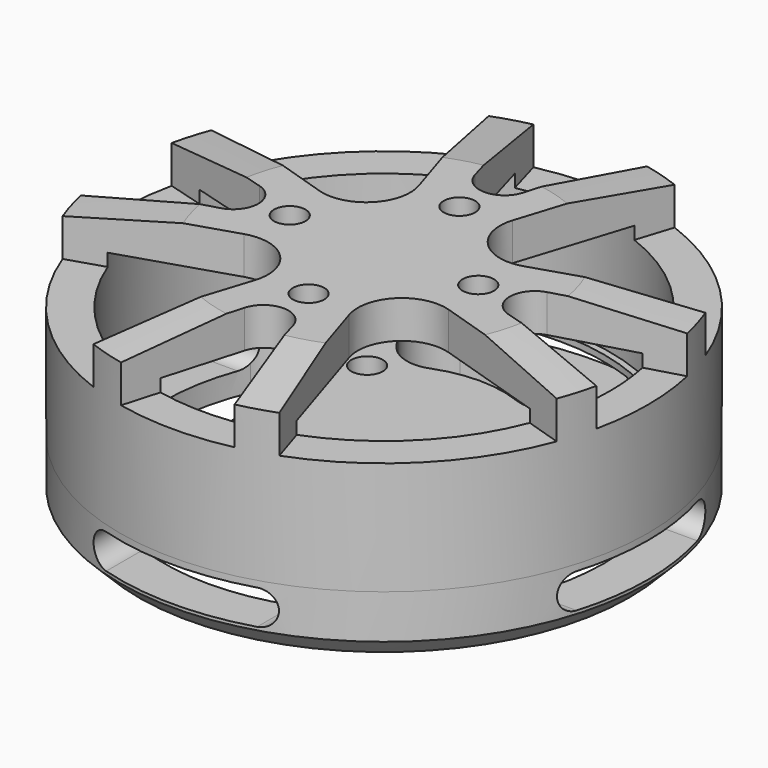
from build123d import *

# Parameters (mm, degrees)
F0_R            = 21
F1_DEPTH        = 5
F3_DEPTH        = 5.001
F4_SIZE         = 1.5
F7_DEPTH        = 10
F7_COPIES_COUNT = 4
F8_DEPTH        = 13
F10_DEPTH       = 4
F11_SIZE2       = 8
F11_SIZE        = 1
F12_R           = 18
F13_DEPTH       = 10
F15_D           = 2.5
F17_D           = 2.5


# Not quite as in the source:
# - a pattern or mirror of a feature is missing from the dataset's text; its kind, count and spacing are read off the source's solid


with BuildPart() as f1:
    # F0 (on Top) → F1 (new body)
    with BuildSketch(Plane.XY):
        Circle(F0_R)
    extrude(amount=-F1_DEPTH)

    # F2 (on face) → F3 (cut, through all)
    with BuildSketch(Plane.XY):
        with BuildLine():
            ThreePointArc((-3.4220516481, 8.8622549342), (0, 9.5), (3.4220516481, 8.8622549342))
            ThreePointArc((3.4220516481, 8.8622549342), (5.3769736461, 8.7910804429), (6.9601556698, 9.9401324464))
            Line((6.9601556698, 9.9401324464), (8.1369050061, 11.6207046655))
            ThreePointArc((8.1369050061, 11.6207046655), (8.5636626177, 14.1668496736), (6.8545072608, 16.1017306589))
            ThreePointArc((6.8545072608, 16.1017306589), (0, 17.5), (-6.8545072608, 16.1017306589))
            ThreePointArc((-6.8545072608, 16.1017306589), (-8.5636626177, 14.1668496736), (-8.1369050061, 11.6207046655))
            Line((-8.1369050061, 11.6207046655), (-6.9601556698, 9.9401324464))
            ThreePointArc((-6.9601556698, 9.9401324464), (-5.3769736461, 8.7910804429), (-3.4220516481, 8.8622549342))
        make_face()
        with BuildLine():
            ThreePointArc((-11.6207046655, 8.1369050061), (-14.1668496736, 8.5636626177), (-16.1017306589, 6.8545072608))
            ThreePointArc((-16.1017306589, 6.8545072608), (-17.5, 0), (-16.1017306589, -6.8545072608))
            ThreePointArc((-16.1017306589, -6.8545072608), (-14.1668496736, -8.5636626177), (-11.6207046655, -8.1369050061))
            Line((-11.6207046655, -8.1369050061), (-9.9401324464, -6.9601556698))
            ThreePointArc((-9.9401324464, -6.9601556698), (-8.7910804429, -5.3769736461), (-8.8622549342, -3.4220516481))
            ThreePointArc((-8.8622549342, -3.4220516481), (-9.5, 0), (-8.8622549342, 3.4220516481))
            ThreePointArc((-8.8622549342, 3.4220516481), (-8.7910804429, 5.3769736461), (-9.9401324464, 6.9601556698))
            Line((-9.9401324464, 6.9601556698), (-11.6207046655, 8.1369050061))
        make_face()
        with BuildLine():
            ThreePointArc((-8.1369050061, -11.6207046655), (-8.5636626177, -14.1668496736), (-6.8545072608, -16.1017306589))
            ThreePointArc((-6.8545072608, -16.1017306589), (0, -17.5), (6.8545072608, -16.1017306589))
            ThreePointArc((6.8545072608, -16.1017306589), (8.5636626177, -14.1668496736), (8.1369050061, -11.6207046655))
            Line((8.1369050061, -11.6207046655), (6.9601556698, -9.9401324464))
            ThreePointArc((6.9601556698, -9.9401324464), (5.3769736461, -8.7910804429), (3.4220516481, -8.8622549342))
            ThreePointArc((3.4220516481, -8.8622549342), (0, -9.5), (-3.4220516481, -8.8622549342))
            ThreePointArc((-3.4220516481, -8.8622549342), (-5.3769736461, -8.7910804429), (-6.9601556698, -9.9401324464))
            Line((-6.9601556698, -9.9401324464), (-8.1369050061, -11.6207046655))
        make_face()
        with BuildLine():
            ThreePointArc((11.6207046655, -8.1369050061), (14.1668496736, -8.5636626177), (16.1017306589, -6.8545072608))
            ThreePointArc((16.1017306589, -6.8545072608), (17.5, 0), (16.1017306589, 6.8545072608))
            ThreePointArc((16.1017306589, 6.8545072608), (14.1668496736, 8.5636626177), (11.6207046655, 8.1369050061))
            Line((11.6207046655, 8.1369050061), (9.9401324464, 6.9601556698))
            ThreePointArc((9.9401324464, 6.9601556698), (8.7910804429, 5.3769736461), (8.8622549342, 3.4220516481))
            ThreePointArc((8.8622549342, 3.4220516481), (9.5, 0), (8.8622549342, -3.4220516481))
            ThreePointArc((8.8622549342, -3.4220516481), (8.7910804429, -5.3769736461), (9.9401324464, -6.9601556698))
            Line((9.9401324464, -6.9601556698), (11.6207046655, -8.1369050061))
        make_face()
    extrude(amount=-F3_DEPTH, mode=Mode.SUBTRACT)

    # F4
    f4_edges = [f1.edges().sort_by_distance(p)[0] for p in [
        (-21, 0, -5),
    ]]
    chamfer(f4_edges, length=F4_SIZE)

    # F6 (on offset) → F7 (cut)
    with BuildSketch(Plane.XZ.offset(25)):
        with BuildLine():
            Line((6, -0.5), (-6, -0.5))
            ThreePointArc((-6, -0.5), (-7.375, -1.875), (-6, -3.25))
            Line((-6, -3.25), (6, -3.25))
            ThreePointArc((6, -3.25), (7.375, -1.875), (6, -0.5))
        make_face()
    f7 = extrude(amount=-F7_DEPTH, mode=Mode.SUBTRACT)

    # F7_copies: F7 ×4 about axis
    f7_copies_axis = Axis((0, 0, 0), (0, 0, 1))
    for i in range(1, F7_COPIES_COUNT):
        add(f7.rotate(f7_copies_axis, i * 360 / F7_COPIES_COUNT), mode=Mode.SUBTRACT)

    # F17 (through all)
    with Locations(Plane(origin=(0, 0, -5), x_dir=(1, 0, 0), z_dir=(0, 0, -1))):
        with Locations((-6.7175144213, -6.7175144213), (-8.8388347648, 8.8388347648), (6.7175144213, 6.7175144213), (8.8388347648, -8.8388347648)):
            Hole(F17_D / 2)


with BuildPart() as f8:
    # F0 (on Top) → F8 (new body)
    with BuildSketch(Plane.XY):
        Circle(F0_R)
    extrude(amount=F8_DEPTH)

    # F9 (on face) → F10 (cut)
    with BuildSketch(Plane.XY.offset(13)):
        with BuildLine():
            Line((-4.5201593688, 20.5077585143), (-1.9225233919, 11.4487252884))
            ThreePointArc((-1.9225233919, 11.4487252884), (0, 10), (1.9225233919, 11.4487252884))
            Line((1.9225233919, 11.4487252884), (4.5201593688, 20.5077585143))
            ThreePointArc((4.5201593688, 20.5077585143), (0, 21), (-4.5201593688, 20.5077585143))
        make_face()
        with BuildLine():
            Line((7.3962318513, 19.6544080145), (3.7353488919, 8.1307749821))
            ThreePointArc((3.7353488919, 8.1307749821), (4.5961940777, 4.5961940777), (8.1307749821, 3.7353488919))
            Line((8.1307749821, 3.7353488919), (19.6544080145, 7.3962318513))
            ThreePointArc((19.6544080145, 7.3962318513), (14.8492424049, 14.8492424049), (7.3962318513, 19.6544080145))
        make_face()
        with BuildLine():
            Line((-20.5077585143, -4.5201593688), (-11.4487252884, -1.9225233919))
            ThreePointArc((-11.4487252884, -1.9225233919), (-10, 0), (-11.4487252884, 1.9225233919))
            Line((-11.4487252884, 1.9225233919), (-20.5077585143, 4.5201593688))
            ThreePointArc((-20.5077585143, 4.5201593688), (-21, 0), (-20.5077585143, -4.5201593688))
        make_face()
        with BuildLine():
            Line((-19.6544080145, 7.3962318513), (-8.1307749821, 3.7353488919))
            ThreePointArc((-8.1307749821, 3.7353488919), (-4.5961940777, 4.5961940777), (-3.7353488919, 8.1307749821))
            Line((-3.7353488919, 8.1307749821), (-7.3962318513, 19.6544080145))
            ThreePointArc((-7.3962318513, 19.6544080145), (-14.8492424049, 14.8492424049), (-19.6544080145, 7.3962318513))
        make_face()
        with BuildLine():
            Line((4.5201593688, -20.5077585143), (1.9225233919, -11.4487252884))
            ThreePointArc((1.9225233919, -11.4487252884), (0, -10), (-1.9225233919, -11.4487252884))
            Line((-1.9225233919, -11.4487252884), (-4.5201593688, -20.5077585143))
            ThreePointArc((-4.5201593688, -20.5077585143), (0, -21), (4.5201593688, -20.5077585143))
        make_face()
        with BuildLine():
            Line((-7.3962318513, -19.6544080145), (-3.7353488919, -8.1307749821))
            ThreePointArc((-3.7353488919, -8.1307749821), (-4.5961940777, -4.5961940777), (-8.1307749821, -3.7353488919))
            Line((-8.1307749821, -3.7353488919), (-19.6544080145, -7.3962318513))
            ThreePointArc((-19.6544080145, -7.3962318513), (-14.8492424049, -14.8492424049), (-7.3962318513, -19.6544080145))
        make_face()
        with BuildLine():
            Line((20.5077585143, 4.5201593688), (11.4487252884, 1.9225233919))
            ThreePointArc((11.4487252884, 1.9225233919), (10, 0), (11.4487252884, -1.9225233919))
            Line((11.4487252884, -1.9225233919), (20.5077585143, -4.5201593688))
            ThreePointArc((20.5077585143, -4.5201593688), (21, 0), (20.5077585143, 4.5201593688))
        make_face()
        with BuildLine():
            Line((19.6544080145, -7.3962318513), (8.1307749821, -3.7353488919))
            ThreePointArc((8.1307749821, -3.7353488919), (4.5961940777, -4.5961940777), (3.7353488919, -8.1307749821))
            Line((3.7353488919, -8.1307749821), (7.3962318513, -19.6544080145))
            ThreePointArc((7.3962318513, -19.6544080145), (14.8492424049, -14.8492424049), (19.6544080145, -7.3962318513))
        make_face()
    extrude(amount=-F10_DEPTH, mode=Mode.SUBTRACT)

    # F11
    f11_edges = [f8.edges().sort_by_distance(p)[0] for p in [
        (-20.132507, -5.973453, 13),
        (-20.132507, 5.973453, 13),
        (-5.973453, 20.132507, 13),
        (5.973453, 20.132507, 13),
        (20.132507, 5.973453, 13),
        (20.132507, -5.973453, 13),
        (5.973453, -20.132507, 13),
        (-5.973453, -20.132507, 13),
    ]]
    chamfer(f11_edges, length=F11_SIZE, length2=F11_SIZE2)

    # F12 (on face) → F13 (cut)
    with BuildSketch(Plane(origin=(0, 0, 0), x_dir=(1, 0, 0), z_dir=(0, 0, -1))):
        Circle(F12_R)
    extrude(amount=-F13_DEPTH, mode=Mode.SUBTRACT)

    # F15 (through all)
    with Locations(Plane.XY.offset(13)):
        with Locations((0, 7.5), (7.5, 0), (0, -7.5), (-7.5, 0)):
            Hole(F15_D / 2)


solid = Compound([f1.part, f8.part])
